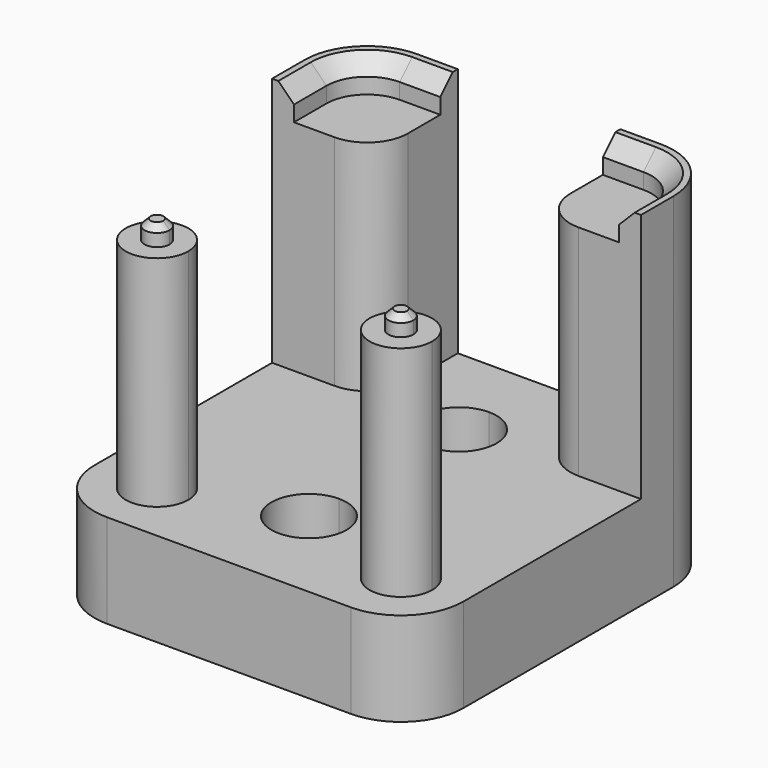
from build123d import *

# Parameters (mm, degrees)
F0_W     = 26
F0_H     = 3.5
F1_DEPTH = 15
F2_DEPTH = 50
F3_DEPTH = 53
F4_DEPTH = 3
F5_DEPTH = 55
F6_SIZE  = 2.5
F7_SIZE  = 1


# Not quite as in the source:
# - a feature names something its author has since deleted; it is built from what else it names


with BuildPart() as f1:
    # F0 (on Top) → F1 (new body)
    with BuildSketch(Plane.XY):
        with Locations((0, 29.25)):
            Rectangle(F0_W, F0_H)
        with BuildLine():
            Line((29.5, -21), (29.5, 14.5))
            Line((29.5, 14.5), (26, 14.5))
            Line((26, 14.5), (19.5, 14.5))
            Line((19.5, 14.5), (19.5, 0))
            Line((19.5, 0), (19.5, -16))
            ThreePointArc((19.5, -16), (23.0355339059, -17.4644660941), (24.5, -21))
            ThreePointArc((24.5, -21), (19.5, -26), (14.5, -21))
            Line((14.5, -21), (0, -21))
            Line((0, -21), (-14.5, -21))
            ThreePointArc((-14.5, -21), (-23.0355339059, -24.5355339059), (-19.5, -16))
            Line((-19.5, -16), (-19.5, 14.5))
            Line((-19.5, 14.5), (-26, 14.5))
            Line((-26, 14.5), (-29.5, 14.5))
            Line((-29.5, 14.5), (-29.5, -21))
            ThreePointArc((-29.5, -21), (-26.5710678119, -28.0710678119), (-19.5, -31))
            Line((-19.5, -31), (19.5, -31))
            ThreePointArc((19.5, -31), (26.5710678119, -28.0710678119), (29.5, -21))
        make_face()
        with BuildLine():
            Line((19.5, 0), (19.5, 14.5))
            Line((19.5, 14.5), (5.9791303716, 14.5))
            ThreePointArc((5.9791303716, 14.5), (4.0620192023, 10.5841195668), (0, 9))
            Line((0, 9), (0, 0))
            Line((0, 0), (19.5, 0))
        make_face()
        with BuildLine():
            Line((-5.9791303716, 14.5), (-19.5, 14.5))
            Line((-19.5, 14.5), (-19.5, -16))
            ThreePointArc((-19.5, -16), (-15.9644660941, -17.4644660941), (-14.5, -21))
            Line((-14.5, -21), (0, -21))
            ThreePointArc((0, -21), (-6, -15), (0, -9))
            Line((0, -9), (0, 0))
            Line((0, 0), (0, 9))
            ThreePointArc((0, 9), (-4.0620192023, 10.5841195668), (-5.9791303716, 14.5))
        make_face()
        with BuildLine():
            Line((19.5, -16), (19.5, 0))
            Line((19.5, 0), (0, 0))
            Line((0, 0), (0, -9))
            ThreePointArc((0, -9), (4.2426406871, -10.7573593129), (6, -15))
            ThreePointArc((6, -15), (4.2426406871, -19.2426406871), (0, -21))
            Line((0, -21), (14.5, -21))
            ThreePointArc((14.5, -21), (15.9644660941, -17.4644660941), (19.5, -16))
        make_face()
        Polygon((13, 21), (13, 27.5), (-13, 27.5), (-13, 21), (0, 21), align=None)
        with BuildLine():
            Line((0, 21), (-13, 21))
            ThreePointArc((-13, 21), (-14.9038059223, 16.4038059223), (-19.5, 14.5))
            Line((-19.5, 14.5), (-5.9791303716, 14.5))
            ThreePointArc((-5.9791303716, 14.5), (-4.4158804332, 19.0620192023), (0, 21))
        make_face()
        with BuildLine():
            ThreePointArc((19.5, 14.5), (14.9038059223, 16.4038059223), (13, 21))
            Line((13, 21), (0, 21))
            ThreePointArc((0, 21), (4.2426406871, 19.2426406871), (6, 15))
            ThreePointArc((6, 15), (5.9947803225, 14.7497823241), (5.9791303716, 14.5))
            Line((5.9791303716, 14.5), (19.5, 14.5))
        make_face()
    extrude(amount=F1_DEPTH)

    # F0 (on Top) → F2 (join)
    with BuildSketch(Plane.XY):
        with BuildLine():
            ThreePointArc((-13, 21), (-14.9038059223, 25.5961940777), (-19.5, 27.5))
            ThreePointArc((-19.5, 27.5), (-24.0961940777, 25.5961940777), (-26, 21))
            ThreePointArc((-26, 21), (-24.0961940777, 16.4038059223), (-19.5, 14.5))
            Line((-19.5, 14.5), (-19.5, 21))
            Line((-19.5, 21), (-13, 21))
        make_face()
        with BuildLine():
            ThreePointArc((-19.5, 14.5), (-14.9038059223, 16.4038059223), (-13, 21))
            Line((-13, 21), (-19.5, 21))
            Line((-19.5, 21), (-19.5, 14.5))
        make_face()
        with BuildLine():
            Line((-13, 21), (-13, 27.5))
            Line((-13, 27.5), (-19.5, 27.5))
            ThreePointArc((-19.5, 27.5), (-14.9038059223, 25.5961940777), (-13, 21))
        make_face()
        with BuildLine():
            ThreePointArc((26, 21), (24.0961940777, 25.5961940777), (19.5, 27.5))
            ThreePointArc((19.5, 27.5), (14.9038059223, 25.5961940777), (13, 21))
            Line((13, 21), (19.5, 21))
            Line((19.5, 21), (19.5, 14.5))
            ThreePointArc((19.5, 14.5), (24.0961940777, 16.4038059223), (26, 21))
        make_face()
        with BuildLine():
            Line((19.5, 21), (13, 21))
            ThreePointArc((13, 21), (14.9038059223, 16.4038059223), (19.5, 14.5))
            Line((19.5, 14.5), (19.5, 21))
        make_face()
        with BuildLine():
            ThreePointArc((24.5, -21), (23.0355339059, -17.4644660941), (19.5, -16))
            Line((19.5, -16), (19.5, -19))
            ThreePointArc((19.5, -19), (20.9142135624, -19.5857864376), (21.5, -21))
            ThreePointArc((21.5, -21), (19.5, -23), (17.5, -21))
            Line((17.5, -21), (14.5, -21))
            ThreePointArc((14.5, -21), (19.5, -26), (24.5, -21))
        make_face()
        with BuildLine():
            Line((19.5, -19), (19.5, -16))
            ThreePointArc((19.5, -16), (15.9644660941, -17.4644660941), (14.5, -21))
            Line((14.5, -21), (17.5, -21))
            ThreePointArc((17.5, -21), (18.0857864376, -19.5857864376), (19.5, -19))
        make_face()
        with BuildLine():
            Line((-19.5, -19), (-19.5, -16))
            ThreePointArc((-19.5, -16), (-23.0355339059, -24.5355339059), (-14.5, -21))
            Line((-14.5, -21), (-17.5, -21))
            ThreePointArc((-17.5, -21), (-20.9142135624, -22.4142135624), (-19.5, -19))
        make_face()
        with BuildLine():
            ThreePointArc((-14.5, -21), (-15.9644660941, -17.4644660941), (-19.5, -16))
            Line((-19.5, -16), (-19.5, -19))
            ThreePointArc((-19.5, -19), (-18.0857864376, -19.5857864376), (-17.5, -21))
            Line((-17.5, -21), (-14.5, -21))
        make_face()
        with BuildLine():
            Line((19.5, 27.5), (13, 27.5))
            Line((13, 27.5), (13, 21))
            ThreePointArc((13, 21), (14.9038059223, 25.5961940777), (19.5, 27.5))
        make_face()
        with BuildLine():
            Line((19.5, 14.5), (26, 14.5))
            Line((26, 14.5), (26, 21))
            ThreePointArc((26, 21), (24.0961940777, 16.4038059223), (19.5, 14.5))
        make_face()
        with BuildLine():
            ThreePointArc((-19.5, 14.5), (-24.0961940777, 16.4038059223), (-26, 21))
            Line((-26, 21), (-26, 14.5))
            Line((-26, 14.5), (-19.5, 14.5))
        make_face()
    extrude(amount=F2_DEPTH)

    # F0 (on Top) → F3 (join)
    with BuildSketch(Plane.XY):
        with BuildLine():
            Line((-19.5, -21), (-19.5, -19))
            ThreePointArc((-19.5, -19), (-20.9142135624, -22.4142135624), (-17.5, -21))
            Line((-17.5, -21), (-19.5, -21))
        make_face()
        with BuildLine():
            ThreePointArc((-17.5, -21), (-18.0857864376, -19.5857864376), (-19.5, -19))
            Line((-19.5, -19), (-19.5, -21))
            Line((-19.5, -21), (-17.5, -21))
        make_face()
        with BuildLine():
            Line((19.5, -21), (19.5, -19))
            ThreePointArc((19.5, -19), (18.0857864376, -19.5857864376), (17.5, -21))
            Line((17.5, -21), (19.5, -21))
        make_face()
        with BuildLine():
            ThreePointArc((21.5, -21), (20.9142135624, -19.5857864376), (19.5, -19))
            Line((19.5, -19), (19.5, -21))
            Line((19.5, -21), (17.5, -21))
            ThreePointArc((17.5, -21), (19.5, -23), (21.5, -21))
        make_face()
    extrude(amount=F3_DEPTH)

    # F0 (on Top) → F4 (join)
    with BuildSketch(Plane.XY):
        with BuildLine():
            Line((-1.6770509831, 14.5), (-5.9791303716, 14.5))
            ThreePointArc((-5.9791303716, 14.5), (-4.0620192023, 10.5841195668), (0, 9))
            Line((0, 9), (0, 13.25))
            ThreePointArc((0, 13.25), (-1.0458250332, 13.59687848), (-1.6770509831, 14.5))
        make_face()
        with BuildLine():
            ThreePointArc((0, 9), (4.0620192023, 10.5841195668), (5.9791303716, 14.5))
            Line((5.9791303716, 14.5), (1.6770509831, 14.5))
            ThreePointArc((1.6770509831, 14.5), (1.0458250332, 13.59687848), (0, 13.25))
            Line((0, 13.25), (0, 9))
        make_face()
        with BuildLine():
            ThreePointArc((6, 15), (4.2426406871, 19.2426406871), (0, 21))
            ThreePointArc((0, 21), (-4.4158804332, 19.0620192023), (-5.9791303716, 14.5))
            Line((-5.9791303716, 14.5), (-1.6770509831, 14.5))
            ThreePointArc((-1.6770509831, 14.5), (-0.2526467688, 16.7316667145), (1.75, 15))
            ThreePointArc((1.75, 15), (1.7316667145, 14.7473532312), (1.6770509831, 14.5))
            Line((1.6770509831, 14.5), (5.9791303716, 14.5))
            ThreePointArc((5.9791303716, 14.5), (5.9947803225, 14.7497823241), (6, 15))
        make_face()
        with BuildLine():
            ThreePointArc((6, -15), (4.2426406871, -10.7573593129), (0, -9))
            ThreePointArc((0, -9), (-6, -15), (0, -21))
            ThreePointArc((0, -21), (4.2426406871, -19.2426406871), (6, -15))
        make_face()
        with BuildLine():
            ThreePointArc((1.75, -15), (-1.2374368671, -16.2374368671), (0, -13.25))
            ThreePointArc((0, -13.25), (1.2374368671, -13.7625631329), (1.75, -15))
        make_face(mode=Mode.SUBTRACT)
    extrude(amount=F4_DEPTH)

    # F0 (on Top) → F5 (join)
    with BuildSketch(Plane.XY):
        with BuildLine():
            ThreePointArc((29.5, 21), (26.5710678119, 28.0710678119), (19.5, 31))
            Line((19.5, 31), (13, 31))
            Line((13, 31), (13, 27.5))
            Line((13, 27.5), (19.5, 27.5))
            ThreePointArc((19.5, 27.5), (24.0961940777, 25.5961940777), (26, 21))
            Line((26, 21), (26, 14.5))
            Line((26, 14.5), (29.5, 14.5))
            Line((29.5, 14.5), (29.5, 21))
        make_face()
        with BuildLine():
            Line((-13, 27.5), (-13, 31))
            Line((-13, 31), (-19.5, 31))
            ThreePointArc((-19.5, 31), (-26.5710678119, 28.0710678119), (-29.5, 21))
            Line((-29.5, 21), (-29.5, 14.5))
            Line((-29.5, 14.5), (-26, 14.5))
            Line((-26, 14.5), (-26, 21))
            ThreePointArc((-26, 21), (-24.0961940777, 25.5961940777), (-19.5, 27.5))
            Line((-19.5, 27.5), (-13, 27.5))
        make_face()
    extrude(amount=F5_DEPTH)

    # F6
    f6_edges = [f1.edges().sort_by_distance(p)[0] for p in [
        (24.096194, 25.596194, 55),
        (16.25, 27.5, 55),
        (-16.25, 27.5, 55),
        (-24.096194, 25.596194, 55),
    ]]
    chamfer(f6_edges, length=F6_SIZE)

    # F7
    f7_edges = [f1.edges().sort_by_distance(p)[0] for p in [
        (-21.5, -21, 53),
        (21.5, -21, 53),
    ]]
    chamfer(f7_edges, length=F7_SIZE)


solid = f1.part
